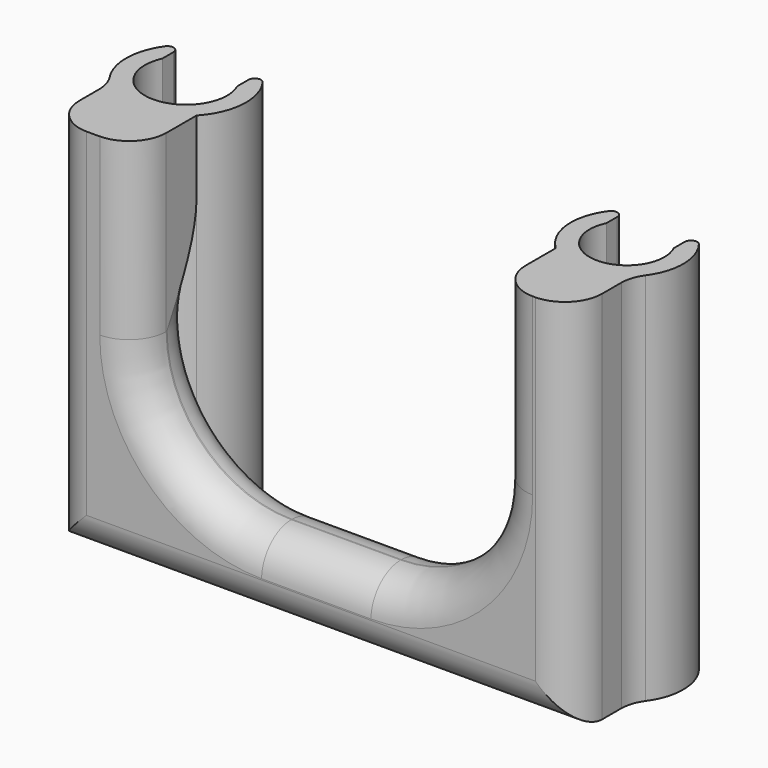
from build123d import *

# Parameters (mm, degrees)
F1_DEPTH     = 30
F0_W         = 28.7549032803
F0_H         = 6
F2_DEPTH     = 6
F3_R         = 10
F4_T1_DEPTH  = 30
F4_T3_DEPTH  = 8.7549032803
F4_T5_DEPTH  = 56.8499252802
F4_T7_DEPTH  = 45.0048285604
F4_T9_DEPTH  = 21.5024142802
F4_T14_ANGLE = 133.0029351346
F4_S15_R     = 4.5
F4_T16_DEPTH = 18
F4_T20_ANGLE = 133.0029351346
F4_S21_R     = 4.8
F4_T22_DEPTH = 18
F4_T24_ANGLE = 90
F4_T26_ANGLE = 90
F5_R         = 1.1999


# Not quite as in the source:
# - a fillet or chamfer that OpenCascade refuses, or shapes differently, is made with other operations: its cross-section is extruded or revolved along the edge and cut away or added
# - a fillet or chamfer is up to 0.001 mm smaller than in the source, because OpenCascade refuses the exact size


with BuildPart() as f1:
    # F0 (on Top) → F1 (new body)
    with BuildSketch(Plane.XY):
        with BuildLine():
            ThreePointArc((-16.1773164054, -3.3), (-18.954612747, -1.7823089045), (-19.1773164054, 1.3747727085))
            Line((-19.1773164054, 1.3747727085), (-19.1773164054, 2.4979991994))
            ThreePointArc((-19.1773164054, 2.4979991994), (-19.5248178351, 2.9741758326), (-20.0842931496, 2.7884642225))
            ThreePointArc((-20.0842931496, 2.7884642225), (-20.9658664058, -0.3313440718), (-19.663001417, -3.3))
            Line((-19.663001417, -3.3), (-16.1773164054, -3.3))
        make_face()
        with BuildLine():
            Line((-12.6916313938, -3.3), (-16.1773164054, -3.3))
            Line((-16.1773164054, -3.3), (-19.663001417, -3.3))
            ThreePointArc((-19.663001417, -3.3), (-16.1773164054, -4.8), (-12.6916313938, -3.3))
        make_face()
        with BuildLine():
            ThreePointArc((-13.1773164054, 1.3747727085), (-13.4000200638, -1.7823089045), (-16.1773164054, -3.3))
            Line((-16.1773164054, -3.3), (-12.6916313938, -3.3))
            ThreePointArc((-12.6916313938, -3.3), (-11.388766405, -0.3313440718), (-12.2703396612, 2.7884642225))
            ThreePointArc((-12.2703396612, 2.7884642225), (-12.8298149757, 2.9741758326), (-13.1773164054, 2.4979991994))
            Line((-13.1773164054, 2.4979991994), (-13.1773164054, 1.3747727085))
        make_face()
        with BuildLine():
            ThreePointArc((-12.6916313938, -3.3), (-16.1773164054, -4.8), (-19.663001417, -3.3))
            Line((-19.663001417, -3.3), (-19.663001417, -9.3))
            Line((-19.663001417, -9.3), (-12.6916313938, -9.3))
            Line((-12.6916313938, -9.3), (-12.6916313938, -3.3))
        make_face()
    extrude(amount=F1_DEPTH)



with BuildPart() as f1b:
    # F0 (on Top) → F1, piece 2 (new body)
    with BuildSketch(Plane.XY):
        with BuildLine():
            ThreePointArc((15.5226835946, 2.7), (14.6408378727, -0.4038055538), (16.0632718864, -3.3))
            Line((16.0632718864, -3.3), (22.1820953027, -3.3))
            ThreePointArc((22.1820953027, -3.3), (23.6045293165, -0.4038055538), (22.7226835946, 2.7))
            ThreePointArc((22.7226835946, 2.7), (22.1645697116, 2.874341649), (21.8226835946, 2.4))
            Line((21.8226835946, 2.4), (21.8226835946, 1.3076696831))
            ThreePointArc((21.8226835946, 1.3076696831), (19.1226835946, -3), (16.4226835946, 1.3076696831))
            Line((16.4226835946, 1.3076696831), (16.4226835946, 2.4))
            ThreePointArc((16.4226835946, 2.4), (16.0807974776, 2.874341649), (15.5226835946, 2.7))
        make_face()
        with BuildLine():
            Line((22.1820953027, -3.3), (16.0632718864, -3.3))
            ThreePointArc((16.0632718864, -3.3), (19.1226835946, -4.5), (22.1820953027, -3.3))
        make_face()
        with BuildLine():
            ThreePointArc((22.1820953027, -3.3), (19.1226835946, -4.5), (16.0632718864, -3.3))
            Line((16.0632718864, -3.3), (16.0632718864, -9.3))
            Line((16.0632718864, -9.3), (22.1820953027, -9.3))
            Line((22.1820953027, -9.3), (22.1820953027, -3.3))
        make_face()
    extrude(amount=F1_DEPTH)


with BuildPart() as f1_1:
    add(f1.part)

    add(f1b.part)  # F2 merges F1b
    # F0 (on Top) → F2 (join)
    with BuildSketch(Plane.XY):
        with BuildLine():
            ThreePointArc((-12.6916313938, -3.3), (-16.1773164054, -4.8), (-19.663001417, -3.3))
            Line((-19.663001417, -3.3), (-19.663001417, -9.3))
            Line((-19.663001417, -9.3), (-12.6916313938, -9.3))
            Line((-12.6916313938, -9.3), (-12.6916313938, -3.3))
        make_face()
        with Locations((1.6858202463, -6.3)):
            Rectangle(F0_W, F0_H)
        with BuildLine():
            ThreePointArc((22.1820953027, -3.3), (19.1226835946, -4.5), (16.0632718864, -3.3))
            Line((16.0632718864, -3.3), (16.0632718864, -9.3))
            Line((16.0632718864, -9.3), (22.1820953027, -9.3))
            Line((22.1820953027, -9.3), (22.1820953027, -3.3))
        make_face()
    extrude(amount=F2_DEPTH)

    # F3
    f3_edges = [f1_1.edges().sort_by_distance(p)[0] for p in [
        (16.063272, -6.3, 6),
        (-12.691631, -6.3, 6),
    ]]
    fillet(f3_edges, radius=F3_R)

    # F4: fillet of radius 3 on 7 edges, made by hand

    # F4_s2 → F4_t1 (join)
    with BuildSketch(Plane.XY):
        with BuildLine():
            ThreePointArc((22.1816953027, -4.420327149), (22.3294674691, -3.4900015654), (22.7582378631, -2.6512535377))
            Line((22.7582378631, -2.6512535377), (22.5156521191, -2.4743461765))
            ThreePointArc((22.5156521191, -2.4743461765), (22.261583156, -2.7902138987), (21.9779713536, -3.079824))
            Line((21.9779713536, -3.079824), (21.8818553027, -3.3))
            ThreePointArc((21.8818553027, -3.3), (21.8818553027, -3.8601635745), (21.8814553027, -4.420327149))
            Line((21.8814553027, -4.420327149), (22.1816953027, -4.420327149))
        make_face()
        with BuildLine():
            ThreePointArc((-20.1683818991, -2.6660000723), (-19.7918275447, -3.4623566946), (-19.662601417, -4.3337220943))
            Line((-19.662601417, -4.3337220943), (-19.362361417, -4.3337220943))
            ThreePointArc((-19.362361417, -4.3337220943), (-19.362761417, -3.8168610471), (-19.362761417, -3.3))
            Line((-19.362761417, -3.3), (-19.4449718195, -3.093585))
            ThreePointArc((-19.4449718195, -3.093585), (-19.6945698662, -2.8065580611), (-19.9187199473, -2.49922787))
            Line((-19.9187199473, -2.49922787), (-20.1683818991, -2.6660000723))
        make_face()
    extrude(amount=F4_T1_DEPTH)

    # F4_s4 → F4_t3 (cut)
    with BuildSketch(Plane.YZ.offset(-2.6916313938)):
        with BuildLine():
            ThreePointArc((-9.3004, 2.9990343146), (-8.4213203436, 5.1213203436), (-6.2990343146, 6.0004))
            Line((-6.2990343146, 6.0004), (-6.2990343146, 6.3005365685))
            ThreePointArc((-6.2990343146, 6.3005365685), (-7.7995171573, 6.3001365685), (-9.3, 6.3001365685))
            Line((-9.3, 6.3001365685), (-9.6001365685, 6))
            ThreePointArc((-9.6001365685, 6), (-9.6001365685, 4.4995171573), (-9.6005365685, 2.9990343146))
            Line((-9.6005365685, 2.9990343146), (-9.3004, 2.9990343146))
        make_face()
        with BuildLine():
            ThreePointArc((-6.3009656854, 6.0004), (-4.1786796564, 5.1213203436), (-3.2996, 2.9990343146))
            Line((-3.2996, 2.9990343146), (-2.9994634315, 2.9990343146))
            ThreePointArc((-2.9994634315, 2.9990343146), (-2.9998634315, 4.4995171573), (-2.9998634315, 6))
            Line((-2.9998634315, 6), (-3.3, 6.3001365685))
            ThreePointArc((-3.3, 6.3001365685), (-4.8004828427, 6.3001365685), (-6.3009656854, 6.3005365685))
            Line((-6.3009656854, 6.3005365685), (-6.3009656854, 6.0004))
        make_face()
    extrude(amount=F4_T3_DEPTH, mode=Mode.SUBTRACT)

    # F4_s6 → F4_t5 (cut)
    with BuildSketch(Plane.YZ.offset(-27.1654156972)):
        with BuildLine():
            ThreePointArc((-9.3004, 3.0009656854), (-8.4213203436, 0.8786796564), (-6.2990343146, -0.0004))
            Line((-6.2990343146, -0.0004), (-6.2990343146, -0.3005365685))
            ThreePointArc((-6.2990343146, -0.3005365685), (-7.7995171573, -0.3001365685), (-9.3, -0.3001365685))
            Line((-9.3, -0.3001365685), (-9.6001365685, 0))
            ThreePointArc((-9.6001365685, 0), (-9.6001365685, 1.5004828427), (-9.6005365685, 3.0009656854))
            Line((-9.6005365685, 3.0009656854), (-9.3004, 3.0009656854))
        make_face()
    extrude(amount=F4_T5_DEPTH, mode=Mode.SUBTRACT)

    # F4_s8 → F4_t7 (cut)
    with BuildSketch(Plane.XY.offset(-7.5024142802)):
        with BuildLine():
            ThreePointArc((-16.6620357316, -9.3004), (-18.7843217606, -8.4213203436), (-19.663401417, -6.2990343146))
            Line((-19.663401417, -6.2990343146), (-19.9635379855, -6.2990343146))
            ThreePointArc((-19.9635379855, -6.2990343146), (-19.9631379855, -7.7995171573), (-19.9631379855, -9.3))
            Line((-19.9631379855, -9.3), (-19.663001417, -9.6001365685))
            ThreePointArc((-19.663001417, -9.6001365685), (-18.1625185743, -9.6001365685), (-16.6620357316, -9.6005365685))
            Line((-16.6620357316, -9.6005365685), (-16.6620357316, -9.3004))
        make_face()
        with BuildLine():
            ThreePointArc((22.1824953027, -6.2990343146), (21.3034156463, -8.4213203436), (19.1811296173, -9.3004))
            Line((19.1811296173, -9.3004), (19.1811296173, -9.6005365685))
            ThreePointArc((19.1811296173, -9.6005365685), (20.68161246, -9.6001365685), (22.1820953027, -9.6001365685))
            Line((22.1820953027, -9.6001365685), (22.4822318713, -9.3))
            ThreePointArc((22.4822318713, -9.3), (22.4822318713, -7.7995171573), (22.4826318713, -6.2990343146))
            Line((22.4826318713, -6.2990343146), (22.1824953027, -6.2990343146))
        make_face()
    extrude(amount=F4_T7_DEPTH, mode=Mode.SUBTRACT)

    # F4_s10 → F4_t9 (cut)
    with BuildSketch(Plane.XY.offset(16)):
        with BuildLine():
            ThreePointArc((19.0642375719, -9.3004), (16.9419515429, -8.4213203436), (16.0628718864, -6.2990343146))
            Line((16.0628718864, -6.2990343146), (15.7627353179, -6.2990343146))
            ThreePointArc((15.7627353179, -6.2990343146), (15.7631353179, -7.7995171573), (15.7631353179, -9.3))
            Line((15.7631353179, -9.3), (16.0632718864, -9.6001365685))
            ThreePointArc((16.0632718864, -9.6001365685), (17.5637547291, -9.6001365685), (19.0642375719, -9.6005365685))
            Line((19.0642375719, -9.6005365685), (19.0642375719, -9.3004))
        make_face()
        with BuildLine():
            ThreePointArc((-15.6925970792, -9.3004), (-13.5703110503, -8.4213203436), (-12.6912313938, -6.2990343146))
            Line((-12.6912313938, -6.2990343146), (-12.3910948253, -6.2990343146))
            ThreePointArc((-12.3910948253, -6.2990343146), (-12.3914948253, -7.7995171573), (-12.3914948253, -9.3))
            Line((-12.3914948253, -9.3), (-12.6916313938, -9.6001365685))
            ThreePointArc((-12.6916313938, -9.6001365685), (-14.1921142365, -9.6001365685), (-15.6925970792, -9.6005365685))
            Line((-15.6925970792, -9.6005365685), (-15.6925970792, -9.3004))
        make_face()
    extrude(amount=F4_T9_DEPTH, mode=Mode.SUBTRACT)


with BuildPart() as f4_tool12:
    # F4_s13 → F4_t14 (revolve)
    with BuildSketch(Plane.YZ.offset(6.0632718864)):
        with BuildLine():
            ThreePointArc((-6.3009656854, 6.0004), (-4.1786796564, 5.1213203436), (-3.2996, 2.9990343146))
            Line((-3.2996, 2.9990343146), (-2.9994634315, 2.9990343146))
            ThreePointArc((-2.9994634315, 2.9990343146), (-2.9998634315, 4.4995171573), (-2.9998634315, 6))
            Line((-2.9998634315, 6), (-3.3, 6.3001365685))
            ThreePointArc((-3.3, 6.3001365685), (-4.8004828427, 6.3001365685), (-6.3009656854, 6.3005365685))
            Line((-6.3009656854, 6.3005365685), (-6.3009656854, 6.0004))
        make_face()
    revolve(axis=Axis((6.0632718864, -3.3, 16), (0, -1, 0)), revolution_arc=F4_T14_ANGLE)

    # F4_s15 → F4_t16 (cut, symmetric)
    with BuildSketch(Plane.XY.offset(13.4)):
        with Locations((19.1226835946, 0)):
            Circle(F4_S15_R)
    extrude(amount=F4_T16_DEPTH, both=True, mode=Mode.SUBTRACT)


with BuildPart() as f1_2:
    add(f1_1.part)

    # F4_t11: cut F4_tool12
    add(f4_tool12.part, mode=Mode.SUBTRACT)


with BuildPart() as f4_tool18:
    # F4_s19 → F4_t20 (revolve)
    with BuildSketch(Plane.YZ.offset(-2.6916313938)):
        with BuildLine():
            ThreePointArc((-6.3009656854, 6.0004), (-4.1786796564, 5.1213203436), (-3.2996, 2.9990343146))
            Line((-3.2996, 2.9990343146), (-2.9994634315, 2.9990343146))
            ThreePointArc((-2.9994634315, 2.9990343146), (-2.9998634315, 4.4995171573), (-2.9998634315, 6))
            Line((-2.9998634315, 6), (-3.3, 6.3001365685))
            ThreePointArc((-3.3, 6.3001365685), (-4.8004828427, 6.3001365685), (-6.3009656854, 6.3005365685))
            Line((-6.3009656854, 6.3005365685), (-6.3009656854, 6.0004))
        make_face()
    revolve(axis=Axis((-2.6916313938, -3.3, 16), (0, 1, 0)), revolution_arc=F4_T20_ANGLE)

    # F4_s21 → F4_t22 (cut, symmetric)
    with BuildSketch(Plane.XY.offset(13.4)):
        with Locations((-16.1773164054, 0)):
            Circle(F4_S21_R)
    extrude(amount=F4_T22_DEPTH, both=True, mode=Mode.SUBTRACT)


with BuildPart() as f1_3:
    add(f1_2.part)

    # F4_t17: cut F4_tool18
    add(f4_tool18.part, mode=Mode.SUBTRACT)

    # F4_s23 → F4_t24 (revolve, cut)
    with BuildSketch(Plane.YZ.offset(-2.6916313938)):
        with BuildLine():
            ThreePointArc((-9.3004, 2.9990343146), (-8.4213203436, 5.1213203436), (-6.2990343146, 6.0004))
            Line((-6.2990343146, 6.0004), (-6.2990343146, 6.3005365685))
            ThreePointArc((-6.2990343146, 6.3005365685), (-7.7995171573, 6.3001365685), (-9.3, 6.3001365685))
            Line((-9.3, 6.3001365685), (-9.6001365685, 6))
            ThreePointArc((-9.6001365685, 6), (-9.6001365685, 4.4995171573), (-9.6005365685, 2.9990343146))
            Line((-9.6005365685, 2.9990343146), (-9.3004, 2.9990343146))
        make_face()
    revolve(axis=Axis((-2.6916313938, -9.3, 16), (0, 1, 0)), revolution_arc=F4_T24_ANGLE, mode=Mode.SUBTRACT)

    # F4_s25 → F4_t26 (revolve, cut)
    with BuildSketch(Plane.YZ.offset(6.0632718864)):
        with BuildLine():
            ThreePointArc((-9.3004, 2.9990343146), (-8.4213203436, 5.1213203436), (-6.2990343146, 6.0004))
            Line((-6.2990343146, 6.0004), (-6.2990343146, 6.3005365685))
            ThreePointArc((-6.2990343146, 6.3005365685), (-7.7995171573, 6.3001365685), (-9.3, 6.3001365685))
            Line((-9.3, 6.3001365685), (-9.6001365685, 6))
            ThreePointArc((-9.6001365685, 6), (-9.6001365685, 4.4995171573), (-9.6005365685, 2.9990343146))
            Line((-9.6005365685, 2.9990343146), (-9.3004, 2.9990343146))
        make_face()
    revolve(axis=Axis((6.0632718864, -9.3, 16), (0, -1, 0)), revolution_arc=F4_T26_ANGLE, mode=Mode.SUBTRACT)

    # F5 (radius 1.2 in the source; OpenCascade refuses exactly that, so slightly less here)
    f5_edges = [f1_3.edges().sort_by_distance(p)[0] for p in [
        (1.68582, -3.3, 0),
    ]]
    fillet(f5_edges, radius=F5_R)


solid = f1_3.part
